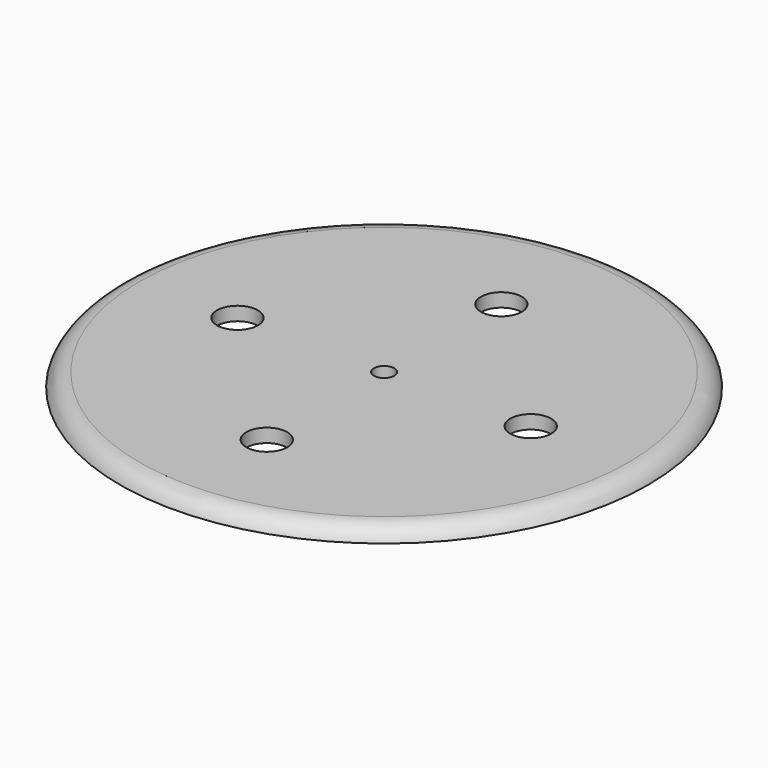
from build123d import *

# Parameters (mm, degrees)
F0_R     = 38.7
F0_R_2   = 3
F0_R_3   = 1.5
F1_DEPTH = 2


# Not quite as in the source:
# - a fillet or chamfer that OpenCascade refuses, or shapes differently, is made with other operations: its cross-section is extruded or revolved along the edge and cut away or added


with BuildPart() as f1:
    # F0 (on Top) → F1 (new body)
    with BuildSketch(Plane.XY):
        Circle(F0_R)
        with Locations((0, -21.5)):
            Circle(F0_R_2, mode=Mode.SUBTRACT)
        with Locations((-21.5, 0)):
            Circle(F0_R_2, mode=Mode.SUBTRACT)
        Circle(F0_R_3, mode=Mode.SUBTRACT)
        with Locations((21.5, 0)):
            Circle(F0_R_2, mode=Mode.SUBTRACT)
        with Locations((0, 21.5)):
            Circle(F0_R_2, mode=Mode.SUBTRACT)
    extrude(amount=F1_DEPTH)

    # F2: fillet of radius 3 on 1 edges, made by hand

    # F2_s1 → F2_t2 (revolve, cut)
    with BuildSketch(Plane.XZ):
        with BuildLine():
            ThreePointArc((38.7, 0), (37.6036236828, 1.4494897428), (35.8715728753, 2))
            Line((35.8715728753, 2), (38.7, 2))
            Line((38.7, 2), (38.7, 0))
        make_face()
    revolve(axis=Axis((0, 0, 2), (0, 0, 1)), mode=Mode.SUBTRACT)


solid = f1.part
